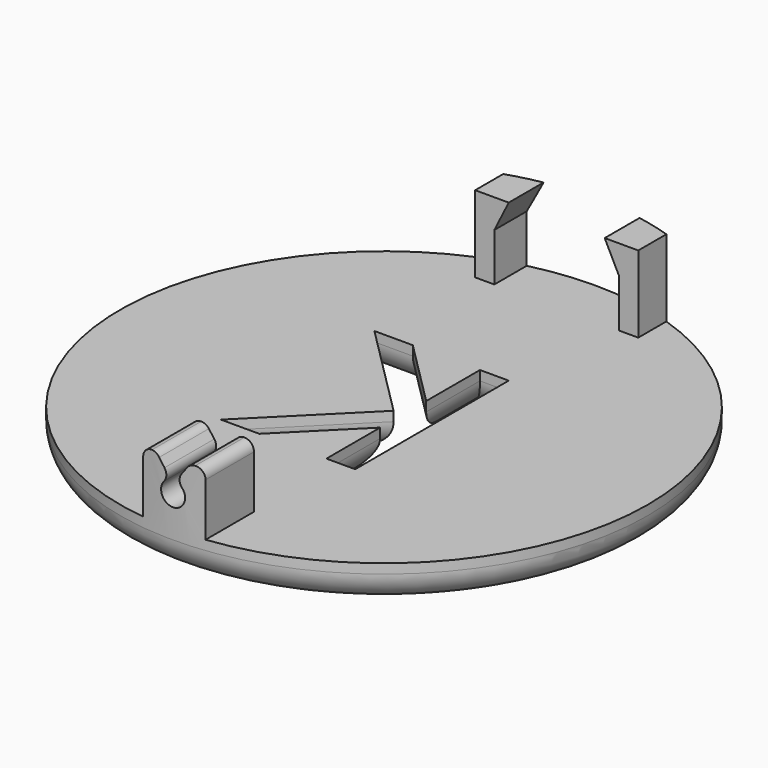
from build123d import *

# Parameters (mm, degrees)
F0_R         = 27.5
F1_DEPTH     = 4
F3_DEPTH     = 8
F4_W         = 13
F4_H         = 5
F5_DEPTH     = 25
F6_W         = 10
F6_H         = 3
F7_DEPTH     = 25
F9_DEPTH     = 25
F11_DEPTH    = 25
F13_DEPTH    = 6.5
F15_D        = 2.5
F17_DEPTH    = 25
F18_T1_DEPTH = 11.8336321238
F19_T1_DEPTH = 11.3072792493
F19_T3_DEPTH = 8.9630793076
F21_DEPTH    = 25
F22_R        = 3


# Not quite as in the source:
# - a fillet or chamfer that OpenCascade refuses, or shapes differently, is made with other operations: its cross-section is extruded or revolved along the edge and cut away or added


with BuildPart() as f1:
    # F0 (on Top) → F1 (new body)
    with BuildSketch(Plane.XY):
        Circle(F0_R)
    extrude(amount=F1_DEPTH)

    # F2 (on face) → F3 (join)
    with BuildSketch(Plane.XY.offset(4)):
        with BuildLine():
            ThreePointArc((8.5, 26.1533936612), (4.3030033163, 27.1612621662), (9e-08, 27.5))
            ThreePointArc((9e-08, 27.5), (-4.3030032274, 27.1612621803), (-8.5, 26.1533936612))
            Line((-8.5, 26.1533936612), (-8.5, 22.5))
            Line((-8.5, 22.5), (8.5, 22.5))
            Line((8.5, 22.5), (8.5, 26.1533936612))
        make_face()
    extrude(amount=F3_DEPTH)

    # F4 (on face) → F5 (cut)
    with BuildSketch(Plane.XZ.offset(-22.5)):
        with Locations((0, 6.5)):
            Rectangle(F4_W, F4_H)
    extrude(amount=-F5_DEPTH, mode=Mode.SUBTRACT)

    # F6 (on face) → F7 (cut)
    with BuildSketch(Plane.XZ.offset(-22.5)):
        with Locations((0, 10.5)):
            Rectangle(F6_W, F6_H)
    extrude(amount=-F7_DEPTH, mode=Mode.SUBTRACT)

    # F8 (on face) → F9 (cut)
    with BuildSketch(Plane.XZ.offset(-22.5)):
        Polygon((-5, 12), (-6.5, 9), (-5, 9), align=None)
    extrude(amount=-F9_DEPTH, mode=Mode.SUBTRACT)

    # F10 (on face) → F11 (cut)
    with BuildSketch(Plane.XZ.offset(-22.5)):
        Polygon((5, 9), (6.5, 9), (5, 12), align=None)
    extrude(amount=-F11_DEPTH, mode=Mode.SUBTRACT)

    # F12 (on face) → F13 (join)
    with BuildSketch(Plane.XY.offset(4)):
        with BuildLine():
            Line((3.25, -27.3072792493), (3.25, -21))
            Line((3.25, -21), (-3.25, -21))
            Line((-3.25, -21), (-3.25, -27.3072792493))
            ThreePointArc((-3.25, -27.3072792493), (-1.627854515, -27.4517775322), (0, -27.5))
            ThreePointArc((0, -27.5), (1.627854515, -27.4517775322), (3.25, -27.3072792493))
        make_face()
    extrude(amount=F13_DEPTH)

    # F15 (through all)
    with Locations(Plane(origin=(0, -21, 0), x_dir=(-1, 0, 0), z_dir=(0, 1, 0))):
        with Locations((0, 7.25)):
            Hole(F15_D / 2)

    # F16 (on face) → F17 (cut)
    with BuildSketch(Plane(origin=(0, -21, 0), x_dir=(-1, 0, 0), z_dir=(0, 1, 0))):
        with BuildLine():
            Line((-1.75, 10.5), (-0.25, 8.4747448714))
            ThreePointArc((-0.25, 8.4747448714), (0, 8.5), (0.25, 8.4747448714))
            Line((0.25, 8.4747448714), (1.75, 10.5))
            Line((1.75, 10.5), (-1.75, 10.5))
        make_face()
    extrude(amount=-F17_DEPTH, mode=Mode.SUBTRACT)

    # F18: fillet of radius 1 on 2 edges, made by hand

    # F18_s2 → F18_t1 (cut)
    with BuildSketch(Plane.XZ.offset(18.3326157402)):
        with BuildLine():
            ThreePointArc((0.8850285779, 9.3321414608), (0.6895138592, 8.6947290379), (0.9381231309, 8.0760901835))
            ThreePointArc((0.9381231309, 8.0760901835), (0.6266103523, 8.331600419), (0.25, 8.4747448714))
            Line((0.25, 8.4747448714), (0.8850285779, 9.3321414608))
        make_face()
        with BuildLine():
            ThreePointArc((-0.9381231309, 8.0760901835), (-0.6895138592, 8.6947290379), (-0.8850285779, 9.3321414608))
            Line((-0.8850285779, 9.3321414608), (-0.25, 8.4747448714))
            ThreePointArc((-0.25, 8.4747448714), (-0.6266103523, 8.331600419), (-0.9381231309, 8.0760901835))
        make_face()
    extrude(amount=F18_T1_DEPTH, mode=Mode.SUBTRACT)

    # F19: fillet of radius 1 on 4 edges, made by hand

    # F19_s2 → F19_t1 (cut)
    with BuildSketch(Plane.XZ.offset(18.5)):
        with BuildLine():
            ThreePointArc((3.25, 9.5), (2.9571067812, 10.2071067812), (2.25, 10.5))
            Line((2.25, 10.5), (3.25, 10.5))
            Line((3.25, 10.5), (3.25, 9.5))
        make_face()
        with BuildLine():
            ThreePointArc((-3.25, 9.5), (-2.9571067812, 10.2071067812), (-2.25, 10.5))
            Line((-2.25, 10.5), (-3.25, 10.5))
            Line((-3.25, 10.5), (-3.25, 9.5))
        make_face()
    extrude(amount=F19_T1_DEPTH, mode=Mode.SUBTRACT)

    # F19_s4 → F19_t3 (cut)
    with BuildSketch(Plane.XZ.offset(19.7405911939)):
        with BuildLine():
            ThreePointArc((2.2537635225, 10.5), (1.8038630505, 10.3930787005), (1.4501704647, 10.0951791306))
            Line((1.4501704647, 10.0951791306), (1.75, 10.5))
            Line((1.75, 10.5), (2.2537635225, 10.5))
        make_face()
        with BuildLine():
            ThreePointArc((-1.4501704647, 10.0951791306), (-1.8038630505, 10.3930787005), (-2.2537635225, 10.5))
            Line((-2.2537635225, 10.5), (-1.75, 10.5))
            Line((-1.75, 10.5), (-1.4501704647, 10.0951791306))
        make_face()
    extrude(amount=F19_T3_DEPTH, mode=Mode.SUBTRACT)

    # F20 (on face) → F21 (cut)
    with BuildSketch(Plane(origin=(0, 0, 0), x_dir=(1, 0, 0), z_dir=(0, 0, -1))):
        Polygon((2, -10), (5, -10), (5, 10), (2, 10), (2, 3), (-5, 10), (-9, 10), (1, 0), (-9, -10), (-5, -10), (2, -3), align=None)
    extrude(amount=-F21_DEPTH, mode=Mode.SUBTRACT)

    # F22
    f22_edges = [f1.edges().sort_by_distance(p)[0] for p in [
        (-27.5, 0, 0),
        (-1.5, 6.5, 0),
        (-7, 10, 0),
        (-4, 5, 0),
        (-4, -5, 0),
        (-7, -10, 0),
        (-1.5, -6.5, 0),
        (2, -6.5, 0),
        (3.5, -10, 0),
        (5, 0, 0),
        (3.5, 10, 0),
        (2, 6.5, 0),
    ]]
    fillet(f22_edges, radius=F22_R)


solid = f1.part
